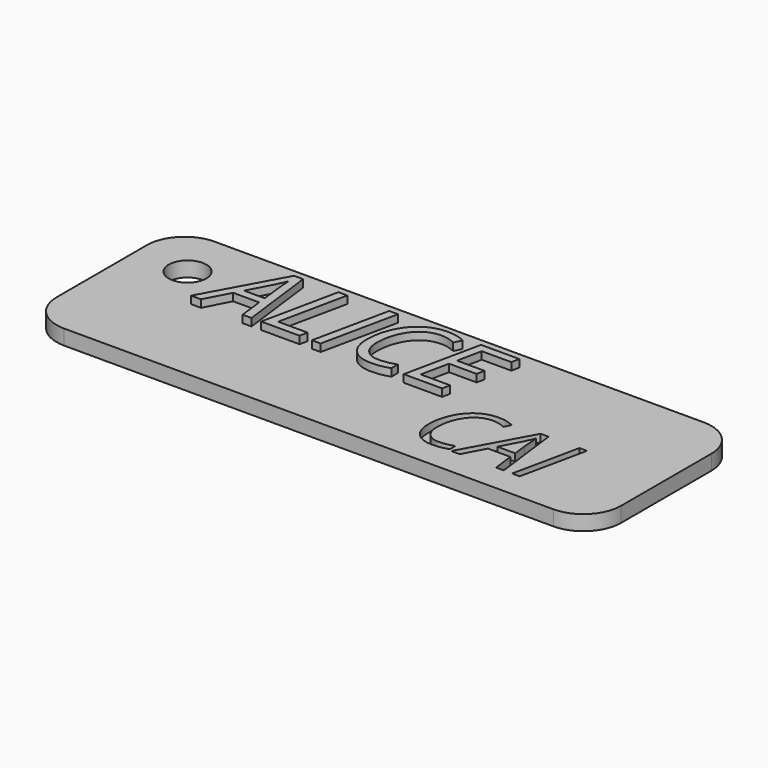
from build123d import *

# Parameters (mm, degrees)
F1_DEPTH     = 2
F3_D         = 5
F4_TEXT_SIZE = 14.221700581
F5_DEPTH     = 3
F6_TEXT_SIZE = 12.3585005187
F7_DEPTH     = 1


# Not quite as in the source:
# - Text() gives the source's letters only with a copy of the font that has no kerning and outlines rounded to 1/6400 em; it was checked with that copy


with BuildPart() as f1:
    # F0 (on Top) → F1 (new body)
    with BuildSketch(Plane.XY):
        with BuildLine():
            Line((32.5, 12.5), (-32.5, 12.5))
            ThreePointArc((-32.5, 12.5), (-36.0355339059, 11.0355339059), (-37.5, 7.5))
            Line((-37.5, 7.5), (-37.5, -7.5))
            ThreePointArc((-37.5, -7.5), (-36.0355339059, -11.0355339059), (-32.5, -12.5))
            Line((-32.5, -12.5), (32.5, -12.5))
            ThreePointArc((32.5, -12.5), (36.0355339059, -11.0355339059), (37.5, -7.5))
            Line((37.5, -7.5), (37.5, 7.5))
            ThreePointArc((37.5, 7.5), (36.0355339059, 11.0355339059), (32.5, 12.5))
        make_face()
    extrude(amount=F1_DEPTH)

    # F3 (through all)
    with Locations(Plane(origin=(0, 0, 0), x_dir=(1, 0, 0), z_dir=(0, 0, -1))):
        with Locations((-30.5, -5.5)):
            Hole(F3_D / 2)

    # F4 (on Top) → F5 (join)
    with BuildSketch(Plane.XY):
        with Locations((-24.8206295073, 0)):
            Text('ALICE', F4_TEXT_SIZE, font='Open Sans', font_style=FontStyle.ITALIC, text_align=(TextAlign.LEFT, TextAlign.BOTTOM))
    extrude(amount=F5_DEPTH)

    # F6 (on face) → F7 (cut)
    with BuildSketch(Plane.XY.offset(2)):
        with Locations((9.5267947763, -8.8981203735)):
            Text('CAI', F6_TEXT_SIZE, font='Open Sans', font_style=FontStyle.ITALIC, text_align=(TextAlign.LEFT, TextAlign.BOTTOM))
    extrude(amount=-F7_DEPTH, mode=Mode.SUBTRACT)


solid = f1.part
